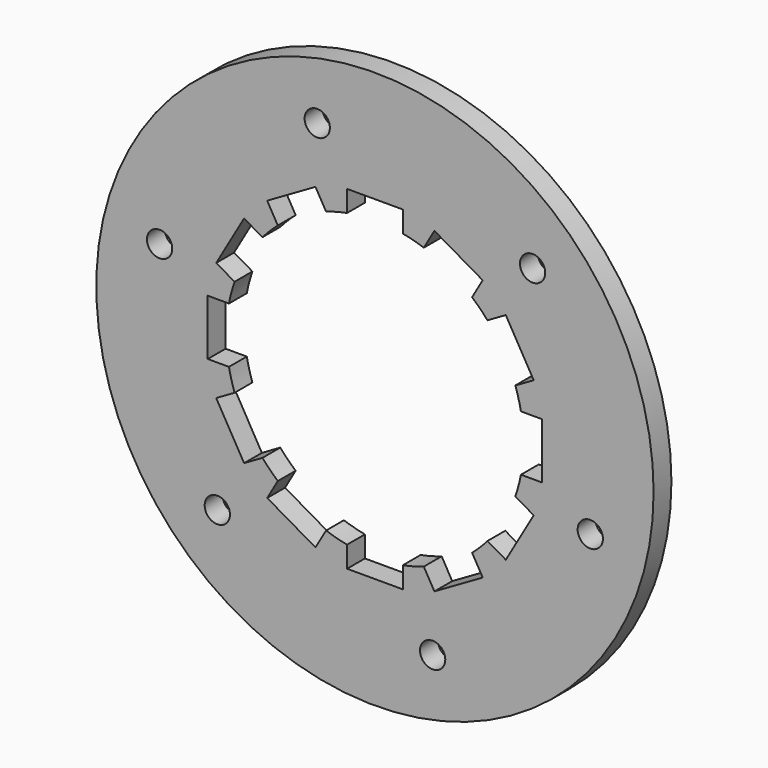
from build123d import *

# Parameters (mm, degrees)
F1_R            = 75
F1_R_2          = 40
F2_DEPTH        = 3
F4_DEPTH        = 35
F4_COPIES_COUNT = 12
F5_R            = 3.4
F6_DEPTH        = 12.5
F6_COPIES_COUNT = 6


# Not quite as in the source:
# - a pattern or mirror of a feature is missing from the dataset's text; its kind, count and spacing are read off the source's solid


with BuildPart() as f2:
    # F1 (on Front) → F2 (new body, symmetric)
    with BuildSketch(Plane.XZ):
        Circle(F1_R)
        Circle(F1_R_2, mode=Mode.SUBTRACT)
    extrude(amount=F2_DEPTH, both=True)

    # F3 (on face) → F4 (cut)
    with BuildSketch(Plane.XZ.offset(3)):
        with BuildLine():
            Line((-7.5, 39.2905841138), (-7.5, 0))
            Line((-7.5, 0), (7.5, 0))
            Line((7.5, 0), (7.5, 39.2905841138))
            ThreePointArc((7.5, 39.2905841138), (0, 40), (-7.5, 39.2905841138))
        make_face()
        with BuildLine():
            Line((-7.5, 45), (-7.5, 39.2905841138))
            ThreePointArc((-7.5, 39.2905841138), (0, 40), (7.5, 39.2905841138))
            Line((7.5, 39.2905841138), (7.5, 45))
            Line((7.5, 45), (-7.5, 45))
        make_face()
    f4 = extrude(amount=-F4_DEPTH, mode=Mode.SUBTRACT)

    # F4_copies: F4 ×12 about axis
    f4_copies_axis = Axis((0, 0, 0), (0, 1, 0))
    for i in range(1, F4_COPIES_COUNT):
        add(f4.rotate(f4_copies_axis, i * 360 / F4_COPIES_COUNT), mode=Mode.SUBTRACT)

    # F5 (on Front) → F6 (cut, symmetric)
    with BuildSketch(Plane.XZ):
        with Locations((42.4264068712, 42.4264068712)):
            Circle(F5_R)
    f6 = extrude(amount=F6_DEPTH, both=True, mode=Mode.SUBTRACT)

    # F6_copies: F6 ×6 about axis
    f6_copies_axis = Axis((0, 0, 0), (0, 1, 0))
    for i in range(1, F6_COPIES_COUNT):
        add(f6.rotate(f6_copies_axis, i * 360 / F6_COPIES_COUNT), mode=Mode.SUBTRACT)


solid = f2.part
